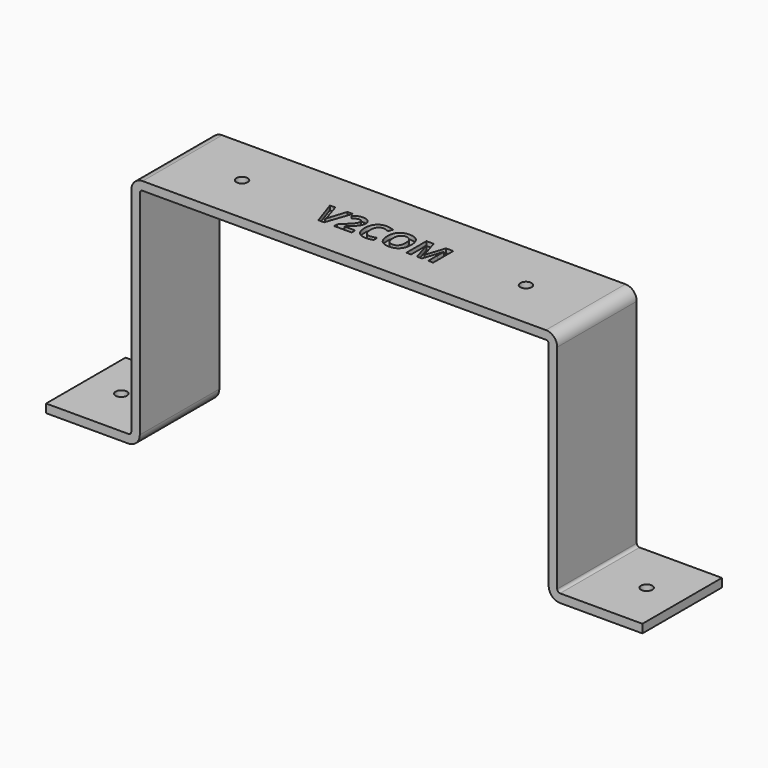
from build123d import *

# Parameters (mm, degrees)
F1_DEPTH     = 35
F2_R         = 2
F3_DEPTH     = 25
F4_R         = 2
F5_DEPTH     = 25
F6_TEXT_SIZE = 12.3895154498
F7_DEPTH     = 1.5


# Not quite as in the source:
# - Text() gives the source's letters only with a copy of the font that has no kerning and outlines rounded to 1/6400 em; it was checked with that copy


with BuildPart() as f1:
    # F0 (on Front) → F1 (new body)
    with BuildSketch(Plane.XZ):
        with BuildLine():
            Line((71, 0), (0, 0))
            Line((0, 0), (0, -3))
            Line((0, -3), (71, -3))
            ThreePointArc((71, -3), (71.7071067812, -3.2928932188), (72, -4))
            Line((72, -4), (72, -79))
            ThreePointArc((72, -79), (73.1715728753, -81.8284271247), (76, -83))
            Line((76, -83), (105, -83))
            Line((105, -83), (105, -80))
            Line((105, -80), (76, -80))
            ThreePointArc((76, -80), (75.2928932188, -79.7071067812), (75, -79))
            Line((75, -79), (75, -4))
            ThreePointArc((75, -4), (73.8284271247, -1.1715728753), (71, 0))
        make_face()
        with BuildLine():
            Line((0, -3), (0, 0))
            Line((0, 0), (-71, 0))
            ThreePointArc((-71, 0), (-73.8284271247, -1.1715728753), (-75, -4))
            Line((-75, -4), (-75, -79))
            ThreePointArc((-75, -79), (-75.2928932188, -79.7071067812), (-76, -80))
            Line((-76, -80), (-105, -80))
            Line((-105, -80), (-105, -83))
            Line((-105, -83), (-76, -83))
            ThreePointArc((-76, -83), (-73.1715728753, -81.8284271247), (-72, -79))
            Line((-72, -79), (-72, -4))
            ThreePointArc((-72, -4), (-71.7071067812, -3.2928932188), (-71, -3))
            Line((-71, -3), (0, -3))
        make_face()
    extrude(amount=F1_DEPTH)

    # F2 (on Top) → F3 (cut)
    with BuildSketch(Plane.XY):
        with Locations((-50, -17.5)):
            Circle(F2_R)
        with Locations((50, -17.5)):
            Circle(F2_R)
    extrude(amount=-F3_DEPTH, mode=Mode.SUBTRACT)

    # F4 (on face) → F5 (cut)
    with BuildSketch(Plane.XY.offset(-80)):
        with Locations((-92.5, -17.5)):
            Circle(F4_R)
        with Locations((92.5, -17.5)):
            Circle(F4_R)
    extrude(amount=-F5_DEPTH, mode=Mode.SUBTRACT)

    # F6 (on face) → F7 (cut)
    with BuildSketch(Plane.XY):
        with Locations((-21.7232730656, -23)):
            Text('V2COM', F6_TEXT_SIZE, font='Open Sans', font_style=FontStyle.BOLD, text_align=(TextAlign.LEFT, TextAlign.BOTTOM))
    extrude(amount=-F7_DEPTH, mode=Mode.SUBTRACT)


solid = f1.part
